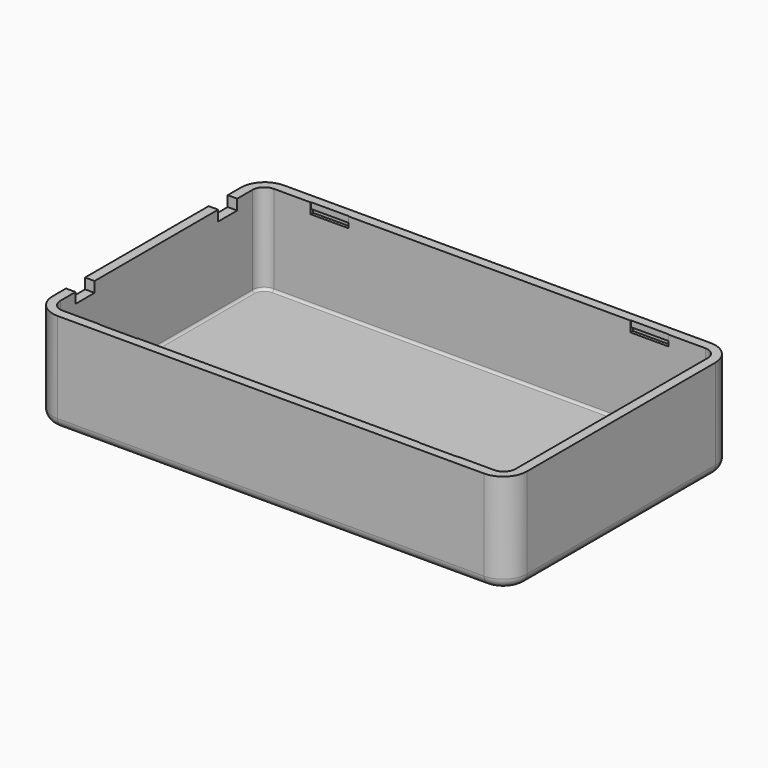
from build123d import *

# Parameters (mm, degrees)
F1_DEPTH = 2
F2_DEPTH = 21
F3_R     = 2
F4_W     = 2
F4_H     = 5
F4_W_2   = 8
F4_H_2   = 0.55
F4_H_3   = 0.1
F5_DEPTH = 2.2
F6_R     = 0.5
F7_DEPTH = 2.9
F8_DEPTH = 1.25


with BuildPart() as f1:
    # F0 (on Top) → F1 (new body)
    with BuildSketch(Plane.XY):
        with BuildLine():
            Line((-44.875, -29.75), (44.875, -29.75))
            ThreePointArc((44.875, -29.75), (48.4105339059, -28.2855339059), (49.875, -24.75))
            Line((49.875, -24.75), (49.875, 24.75))
            ThreePointArc((49.875, 24.75), (48.4105339059, 28.2855339059), (44.875, 29.75))
            Line((44.875, 29.75), (-44.875, 29.75))
            ThreePointArc((-44.875, 29.75), (-48.4105339059, 28.2855339059), (-49.875, 24.75))
            Line((-49.875, 24.75), (-49.875, -24.75))
            ThreePointArc((-49.875, -24.75), (-48.4105339059, -28.2855339059), (-44.875, -29.75))
        make_face()
        with BuildLine():
            ThreePointArc((47.875, -25.25), (47.142766953, -27.017766953), (45.375, -27.75))
            Line((45.375, -27.75), (-45.375, -27.75))
            ThreePointArc((-45.375, -27.75), (-47.142766953, -27.017766953), (-47.875, -25.25))
            Line((-47.875, -25.25), (-47.875, 25.25))
            ThreePointArc((-47.875, 25.25), (-47.142766953, 27.017766953), (-45.375, 27.75))
            Line((-45.375, 27.75), (45.375, 27.75))
            ThreePointArc((45.375, 27.75), (47.142766953, 27.017766953), (47.875, 25.25))
            Line((47.875, 25.25), (47.875, -25.25))
        make_face(mode=Mode.SUBTRACT)
        with BuildLine():
            Line((-45.375, -27.75), (45.375, -27.75))
            ThreePointArc((45.375, -27.75), (47.142766953, -27.017766953), (47.875, -25.25))
            Line((47.875, -25.25), (47.875, 25.25))
            ThreePointArc((47.875, 25.25), (47.142766953, 27.017766953), (45.375, 27.75))
            Line((45.375, 27.75), (-45.375, 27.75))
            ThreePointArc((-45.375, 27.75), (-47.142766953, 27.017766953), (-47.875, 25.25))
            Line((-47.875, 25.25), (-47.875, -25.25))
            ThreePointArc((-47.875, -25.25), (-47.142766953, -27.017766953), (-45.375, -27.75))
        make_face()
    extrude(amount=F1_DEPTH)

    # F0 (on Top) → F2 (join)
    with BuildSketch(Plane.XY):
        with BuildLine():
            Line((-44.875, -29.75), (44.875, -29.75))
            ThreePointArc((44.875, -29.75), (48.4105339059, -28.2855339059), (49.875, -24.75))
            Line((49.875, -24.75), (49.875, 24.75))
            ThreePointArc((49.875, 24.75), (48.4105339059, 28.2855339059), (44.875, 29.75))
            Line((44.875, 29.75), (-44.875, 29.75))
            ThreePointArc((-44.875, 29.75), (-48.4105339059, 28.2855339059), (-49.875, 24.75))
            Line((-49.875, 24.75), (-49.875, -24.75))
            ThreePointArc((-49.875, -24.75), (-48.4105339059, -28.2855339059), (-44.875, -29.75))
        make_face()
        with BuildLine():
            ThreePointArc((47.875, -25.25), (47.142766953, -27.017766953), (45.375, -27.75))
            Line((45.375, -27.75), (-45.375, -27.75))
            ThreePointArc((-45.375, -27.75), (-47.142766953, -27.017766953), (-47.875, -25.25))
            Line((-47.875, -25.25), (-47.875, 25.25))
            ThreePointArc((-47.875, 25.25), (-47.142766953, 27.017766953), (-45.375, 27.75))
            Line((-45.375, 27.75), (45.375, 27.75))
            ThreePointArc((45.375, 27.75), (47.142766953, 27.017766953), (47.875, 25.25))
            Line((47.875, 25.25), (47.875, -25.25))
        make_face(mode=Mode.SUBTRACT)
    extrude(amount=F2_DEPTH)

    # F3
    f3_edges = [f1.edges().sort_by_distance(p)[0] for p in [
        (0, -29.75, 0),
        (-48.410534, -28.285534, 0),
        (-49.875, 0, 0),
        (-48.410534, 28.285534, 0),
        (0, 29.75, 0),
        (48.410534, 28.285534, 0),
        (49.875, 0, 0),
        (48.410534, -28.285534, 0),
    ]]
    fillet(f3_edges, radius=F3_R)

    # F4 (on face) → F5 (cut)
    with BuildSketch(Plane.XY.offset(21)):
        with Locations((-48.875, -18.75)):
            Rectangle(F4_W, F4_H)
        with Locations((-48.875, 18.75)):
            Rectangle(F4_W, F4_H)
        with Locations((-33.625, 28.125)):
            Rectangle(F4_W_2, F4_H_2)
        with Locations((-33.625, 27.8)):
            Rectangle(F4_W_2, F4_H_3)
        with Locations((33.625, 28.125)):
            Rectangle(F4_W_2, F4_H_2)
        with Locations((33.625, 27.8)):
            Rectangle(F4_W_2, F4_H_3)
    extrude(amount=-F5_DEPTH, mode=Mode.SUBTRACT)

    # F6
    f6_edges = [f1.edges().sort_by_distance(p)[0] for p in [
        (47.142767, 27.017767, 2),
        (47.875, 0, 2),
        (47.142767, -27.017767, 2),
        (0, -27.75, 2),
        (-47.142767, -27.017767, 2),
        (-47.875, 0, 2),
        (-47.142767, 27.017767, 2),
        (0, 27.75, 2),
    ]]
    fillet(f6_edges, radius=F6_R)

    # F4 (on face) → F7 (cut)
    with BuildSketch(Plane.XY.offset(21)):
        with Locations((-33.625, -28.125)):
            Rectangle(F4_W_2, F4_H_2)
        with Locations((-33.625, -27.8)):
            Rectangle(F4_W_2, F4_H_3)
        with Locations((33.625, -27.8)):
            Rectangle(F4_W_2, F4_H_3)
        with Locations((33.625, -28.125)):
            Rectangle(F4_W_2, F4_H_2)
    extrude(amount=-F7_DEPTH, mode=Mode.SUBTRACT)

    # F4 (on face) → F8 (join)
    with BuildSketch(Plane.XY.offset(21)):
        with Locations((33.625, 28.125)):
            Rectangle(F4_W_2, F4_H_2)
        with Locations((-33.625, 28.125)):
            Rectangle(F4_W_2, F4_H_2)
        with Locations((-33.625, -28.125)):
            Rectangle(F4_W_2, F4_H_2)
        with Locations((33.625, -28.125)):
            Rectangle(F4_W_2, F4_H_2)
    extrude(amount=-F8_DEPTH)


solid = f1.part
